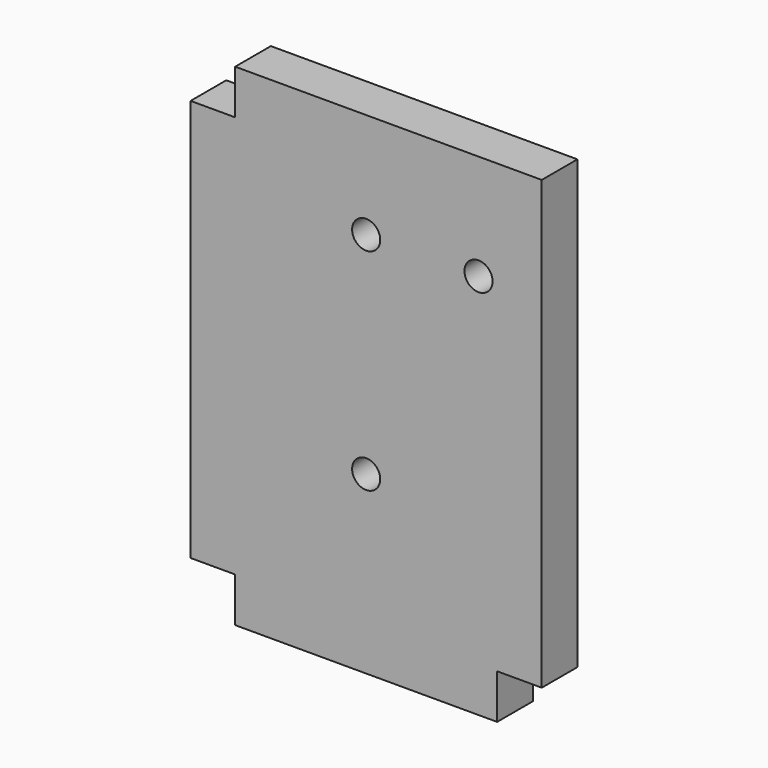
from build123d import *

# Parameters (mm, degrees)
F0_R     = 2
F1_DEPTH = 6.35


# Not quite as in the source:
# - a length typed as a fraction of an inch, garbled in the dataset ("3 / 203.2 mm" for 3/8 in), is restored


with BuildPart() as f1:
    # F0 (on Front) → F1 (new body)
    with BuildSketch(Plane.XZ):
        Polygon((25, 45), (-18.65, 45), (-18.65, 38.65), (-25, 38.65), (-25, 30), (-25, -18.65), (-18.65, -18.65), (-18.65, -25), (18.65, -25), (18.65, -18.65), (25, -18.65), align=None)
        Circle(F0_R, mode=Mode.SUBTRACT)
        with Locations((0, 30)):
            Circle(F0_R, mode=Mode.SUBTRACT)
        with Locations((16, 30)):
            Circle(F0_R, mode=Mode.SUBTRACT)
    extrude(amount=F1_DEPTH)


solid = f1.part
